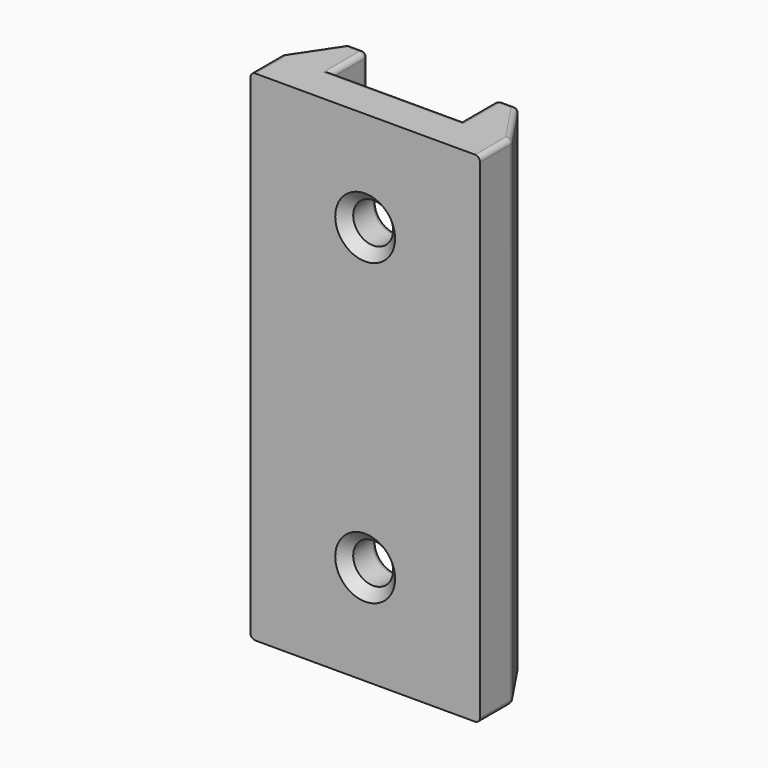
from build123d import *

# Parameters (mm, degrees)
F0_W           = 12
F0_H           = 50
F0_R           = 2
F0_W_2         = 0.5
F0_W_3         = 5
F1_DEPTH       = 4
F2_DEPTH       = 8.5
F3_SIZE2       = 3
F3_SIZE        = 4.5
F4_SIZE2       = 3
F4_SIZE        = 4.5
F5_D           = 4
F5_CSINK_D     = 6
F5_CSINK_ANGLE = 90
F6_R           = 0.5


with BuildPart() as f1:
    # F0 (on Front) → F1 (new body)
    with BuildSketch(Plane.XZ):
        Rectangle(F0_W, F0_H)
        with Locations((0, -15)):
            Circle(F0_R, mode=Mode.SUBTRACT)
        with Locations((0, 15)):
            Circle(F0_R, mode=Mode.SUBTRACT)
        with Locations((6.25, 0)):
            Rectangle(F0_W_2, F0_H)
        with Locations((-6.25, 0)):
            Rectangle(F0_W_2, F0_H)
        with Locations((9, 0)):
            Rectangle(F0_W_3, F0_H)
        with Locations((-9, 0)):
            Rectangle(F0_W_3, F0_H)
    extrude(amount=-F1_DEPTH)

    # F0 (on Front) → F2 (join)
    with BuildSketch(Plane.XZ):
        with Locations((-9, 0)):
            Rectangle(F0_W_3, F0_H)
        with Locations((9, 0)):
            Rectangle(F0_W_3, F0_H)
    extrude(amount=-F2_DEPTH)

    # F3
    f3_edges = [f1.edges().sort_by_distance(p)[0] for p in [
        (-11.5, 8.5, 0),
    ]]
    f3_side = f1.faces().sort_by_distance((-11.5, 4.25, 0))[0]
    chamfer(f3_edges, length=F3_SIZE, length2=F3_SIZE2, reference=f3_side)

    # F4
    f4_edges = [f1.edges().sort_by_distance(p)[0] for p in [
        (11.5, 8.5, 0),
    ]]
    f4_side = f1.faces().sort_by_distance((11.5, 4.25, 0))[0]
    chamfer(f4_edges, length=F4_SIZE, length2=F4_SIZE2, reference=f4_side)

    # F5 (through all)
    with Locations(Plane.XZ):
        with Locations((0, 15), (0, -15)):
            CounterSinkHole(F5_D / 2, F5_CSINK_D / 2, counter_sink_angle=F5_CSINK_ANGLE)

    # F6
    f6_edges = [f1.edges().sort_by_distance(p)[0] for p in [
        (10, 6.25, -25),
        (11.5, 4, 0),
        (8.5, 8.5, 0),
        (10, 6.25, 25),
        (7.5, 8.5, -25),
        (6.5, 8.5, 0),
        (7.5, 8.5, 25),
        (-7.5, 8.5, -25),
        (-8.5, 8.5, 0),
        (-6.5, 8.5, 0),
        (-7.5, 8.5, 25),
        (-10, 6.25, 25),
        (-11.5, 4, 0),
        (-10, 6.25, -25),
        (-2, 4, -15),
        (-2, 4, 15),
        (0, 4, -25),
        (6.5, 6.25, -25),
        (-6.5, 6.25, -25),
        (-11.5, 2, -25),
        (11.5, 2, -25),
        (11.5, 2, 25),
        (6.5, 6.25, 25),
        (0, 4, 25),
        (-6.5, 6.25, 25),
        (-11.5, 2, 25),
    ]]
    fillet(f6_edges, radius=F6_R)


solid = f1.part
